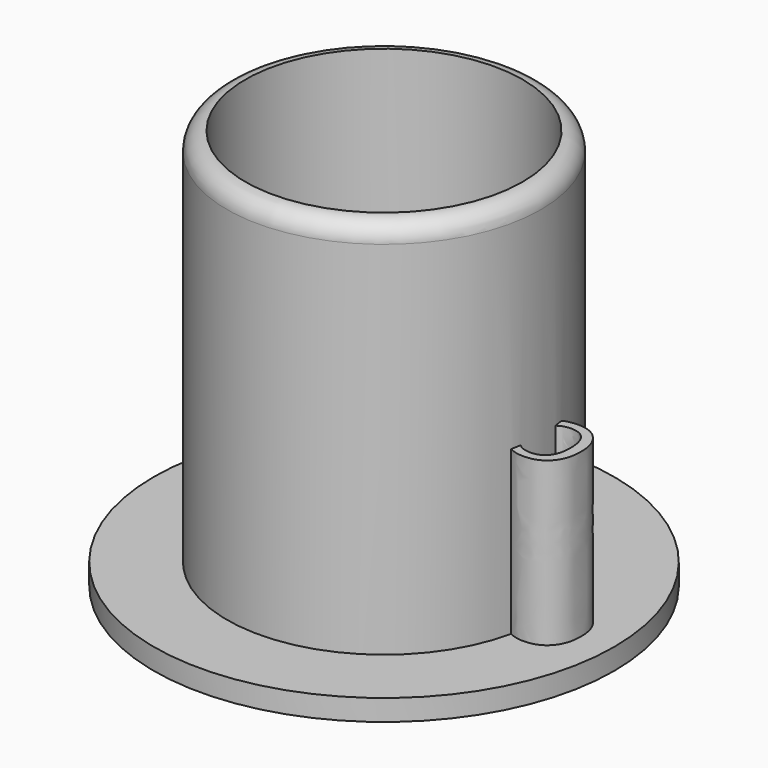
from build123d import *

# Parameters (mm, degrees)
F0_R     = 43.4000447198
F1_DEPTH = 110.744
F2_T     = -5.08
F3_R     = 63.6187489092
F4_DEPTH = 5.842
F5_R     = 5.07999
F6_W     = 2.7671808675
F6_H     = 25.928324776
F7_DEPTH = 50.8


# Not quite as in the source:
# - a fillet or chamfer is up to 0.001 mm smaller than in the source, because OpenCascade refuses the exact size


with BuildPart() as f1:
    # F0 (on Top) → F1 (new body)
    with BuildSketch(Plane.XY):
        Circle(F0_R)
    extrude(amount=F1_DEPTH)

    # F2
    f2_openings = [f1.faces().sort_by_distance(p)[0] for p in [
        (0, 0, 110.744),
    ]]
    offset(amount=F2_T, openings=f2_openings)

    # F3 (on Top) → F4 (join)
    with BuildSketch(Plane.XY):
        Circle(F3_R)
    extrude(amount=F4_DEPTH)

    # F5 (radius 5.08 in the source; OpenCascade refuses exactly that, so slightly less here)
    f5_edges = [f1.edges().sort_by_distance(p)[0] for p in [
        (-43.400045, 0, 110.744),
    ]]
    fillet(f5_edges, radius=F5_R)

    # F6 (on Top) → F7 (join)
    with BuildSketch(Plane.XY):
        with BuildLine():
            ThreePointArc((22.0028883346, -9.7789997235), (23.5536000152, -4.9983854371), (24.0781214104, 0))
            ThreePointArc((24.0781214104, 0), (23.5424460635, 5.0506597592), (21.9592547789, 9.8765915281))
            Line((21.9592547789, 9.8765915281), (21.9592547789, -9.7789997235))
            Line((21.9592547789, -9.7789997235), (22.0028883346, -9.7789997235))
        make_face()
        with BuildLine():
            ThreePointArc((21.9592547789, 9.8765915281), (23.5424460635, 5.0506597592), (24.0781214104, 0))
            ThreePointArc((24.0781214104, 0), (23.5536000152, -4.9983854371), (22.0028883346, -9.7789997235))
            Line((22.0028883346, -9.7789997235), (24.7264356464, -9.7789997235))
            Line((24.7264356464, -9.7789997235), (24.7264356464, 16.1493250525))
            Line((24.7264356464, 16.1493250525), (21.9592547789, 16.1493250525))
            Line((21.9592547789, 16.1493250525), (21.9592547789, 9.8765915281))
        make_face()
        with BuildLine():
            Line((21.9592547789, -9.7789997235), (21.9592547789, 9.8765915281))
            ThreePointArc((21.9592547789, 9.8765915281), (2.7373131328, 23.9220201377), (-19.1605677938, 14.5817890698))
            Line((-19.1605677938, 14.5817890698), (-19.1165860754, 14.5817890698))
            Line((-19.1165860754, 14.5817890698), (-19.1165860754, 4.2168572654))
            Line((-19.1165860754, 4.2168572654), (-6.283051686, 4.2168572654))
            Line((-6.283051686, 4.2168572654), (-6.283051686, 14.5817890698))
            Line((-6.283051686, 14.5817890698), (-3.4518897579, 14.5817890698))
            Line((-3.4518897579, 14.5817890698), (-3.4518897579, -9.7789997235))
            Line((-3.4518897579, -9.7789997235), (-6.283051686, -9.7789997235))
            Line((-6.283051686, -9.7789997235), (-6.283051686, 1.6842736198))
            Line((-6.283051686, 1.6842736198), (-19.1165860754, 1.6842736198))
            Line((-19.1165860754, 1.6842736198), (-19.1165860754, -9.7789997235))
            Line((-19.1165860754, -9.7789997235), (-21.9477480035, -9.7789997235))
            Line((-21.9477480035, -9.7789997235), (-21.9477480035, 9.9021355389))
            ThreePointArc((-21.9477480035, 9.9021355389), (-9.8406062526, -21.9754044158), (22.0028883346, -9.7789997235))
            Line((22.0028883346, -9.7789997235), (21.9592547789, -9.7789997235))
        make_face()
        with BuildLine():
            add(Edge.make_bspline(
                [(13.6843709515, -9.837649029), (12.3780909659, -10.1149002912), (10.5279719658, -10.1149002912)],
                knots=[0, 0, 0, 1, 1, 1], degree=2))
            add(Edge.make_bspline(
                [(10.5279719658, -10.1149002912), (6.4811698879, -10.1149002912), (4.1378635463, -7.6462977061)],
                knots=[0, 0, 0, 1, 1, 1], degree=2))
            add(Edge.make_bspline(
                [(4.1378635463, -7.6462977061), (1.7945572048, -5.177695121), (1.7945572048, -0.8003242304)],
                knots=[0, 0, 0, 1, 1, 1], degree=2))
            add(Edge.make_bspline(
                [(1.7945572048, -0.8003242304), (1.7945572048, 3.6197007006), (3.9699132625, 6.2189312842)],
                knots=[0, 0, 0, 1, 1, 1], degree=2))
            add(Edge.make_bspline(
                [(3.9699132625, 6.2189312842), (6.1452693202, 8.8181618679), (9.81351679, 8.8181618679)],
                knots=[0, 0, 0, 1, 1, 1], degree=2))
            add(Edge.make_bspline(
                [(9.81351679, 8.8181618679), (13.2418352829, 8.8181618679), (15.2412434242, 6.560163607)],
                knots=[0, 0, 0, 1, 1, 1], degree=2))
            add(Edge.make_bspline(
                [(15.2412434242, 6.560163607), (17.2406515655, 4.3021653461), (17.2406515655, 0.601927346)],
                knots=[0, 0, 0, 1, 1, 1], degree=2))
            Line((17.2406515655, 0.601927346), (17.2406515655, -1.1468883082))
            Line((17.2406515655, -1.1468883082), (4.6630414181, -1.1468883082))
            add(Edge.make_bspline(
                [(4.6630414181, -1.1468883082), (4.7483494988, -4.3619365994), (6.2892267063, -6.0281100505)],
                knots=[0, 0, 0, 1, 1, 1], degree=2))
            add(Edge.make_bspline(
                [(6.2892267063, -6.0281100505), (7.8301039139, -7.6942835015), (10.6292753117, -7.6942835015)],
                knots=[0, 0, 0, 1, 1, 1], degree=2))
            add(Edge.make_bspline(
                [(10.6292753117, -7.6942835015), (13.5777358507, -7.6942835015), (16.4568835741, -6.4626480865)],
                knots=[0, 0, 0, 1, 1, 1], degree=2))
            Line((16.4568835741, -6.4626480865), (16.4568835741, -8.9312506716))
            add(Edge.make_bspline(
                [(16.4568835741, -8.9312506716), (14.9906509372, -9.5603977667), (13.6843709515, -9.837649029)],
                knots=[0, 0, 0, 1, 1, 1], degree=2))
        make_face(mode=Mode.SUBTRACT)
        with BuildLine():
            Line((-19.1165860754, 14.5817890698), (-19.1605677938, 14.5817890698))
            ThreePointArc((-19.1605677938, 14.5817890698), (-20.6869088124, 12.3210281406), (-21.9477480035, 9.9021355389))
            Line((-21.9477480035, 9.9021355389), (-21.9477480035, -9.7789997235))
            Line((-21.9477480035, -9.7789997235), (-19.1165860754, -9.7789997235))
            Line((-19.1165860754, -9.7789997235), (-19.1165860754, 1.6842736198))
            Line((-19.1165860754, 1.6842736198), (-6.283051686, 1.6842736198))
            Line((-6.283051686, 1.6842736198), (-6.283051686, -9.7789997235))
            Line((-6.283051686, -9.7789997235), (-3.4518897579, -9.7789997235))
            Line((-3.4518897579, -9.7789997235), (-3.4518897579, 14.5817890698))
            Line((-3.4518897579, 14.5817890698), (-6.283051686, 14.5817890698))
            Line((-6.283051686, 14.5817890698), (-6.283051686, 4.2168572654))
            Line((-6.283051686, 4.2168572654), (-19.1165860754, 4.2168572654))
            Line((-19.1165860754, 4.2168572654), (-19.1165860754, 14.5817890698))
        make_face()
        with BuildLine():
            ThreePointArc((-21.9477480035, 9.9021355389), (-20.6869088124, 12.3210281406), (-19.1605677938, 14.5817890698))
            Line((-19.1605677938, 14.5817890698), (-21.9477480035, 14.5817890698))
            Line((-21.9477480035, 14.5817890698), (-21.9477480035, 9.9021355389))
        make_face()
        with Locations((31.9749566279, 3.1851626645)):
            Rectangle(F6_W, F6_H)
        with BuildLine():
            add(Edge.make_bspline(
                [(54.9841455177, -0.629708069), (54.9841455177, -5.0977187954), (52.7368107669, -7.6063095433)],
                knots=[0, 0, 0, 1, 1, 1], degree=2))
            add(Edge.make_bspline(
                [(52.7261472568, 6.2669170796), (54.9841455177, 3.7156722913), (54.9841455177, -0.629708069)],
                knots=[0, 0, 0, 1, 1, 1], degree=2))
            add(Edge.make_bspline(
                [(46.6399488748, 8.8181618679), (50.4681489959, 8.8181618679), (52.7261472568, 6.2669170796)],
                knots=[0, 0, 0, 1, 1, 1], degree=2))
            add(Edge.make_bspline(
                [(40.4391177593, 6.3255663851), (42.6731231225, 8.8181618679), (46.6399488748, 8.8181618679)],
                knots=[0, 0, 0, 1, 1, 1], degree=2))
            add(Edge.make_bspline(
                [(38.2051123961, -0.629708069), (38.2051123961, 3.8329709023), (40.4391177593, 6.3255663851)],
                knots=[0, 0, 0, 1, 1, 1], degree=2))
            add(Edge.make_bspline(
                [(39.2394728745, -5.66288483), (38.2051123961, -3.5141875475), (38.2051123961, -0.629708069)],
                knots=[0, 0, 0, 1, 1, 1], degree=2))
            add(Edge.make_bspline(
                [(42.1719381484, -8.9632412019), (40.2738333529, -7.8115821125), (39.2394728745, -5.66288483)],
                knots=[0, 0, 0, 1, 1, 1], degree=2))
            add(Edge.make_bspline(
                [(46.5226502638, -10.1149002912), (44.0700429438, -10.1149002912), (42.1719381484, -8.9632412019)],
                knots=[0, 0, 0, 1, 1, 1], degree=2))
            add(Edge.make_bspline(
                [(52.7368107669, -7.6063095433), (50.4894760161, -10.1149002912), (46.5226502638, -10.1149002912)],
                knots=[0, 0, 0, 1, 1, 1], degree=2))
        make_face()
        with BuildLine():
            add(Edge.make_bspline(
                [(41.0735966094, -0.629708069), (41.0735966094, -4.1326711325), (42.4731823083, -5.9641289899)],
                knots=[0, 0, 0, 1, 1, 1], degree=2))
            add(Edge.make_bspline(
                [(42.4571870432, 4.6833858317), (41.0735966094, 2.8999137697), (41.0735966094, -0.629708069)],
                knots=[0, 0, 0, 1, 1, 1], degree=2))
            add(Edge.make_bspline(
                [(46.5546407941, 6.4668578937), (43.840777477, 6.4668578937), (42.4571870432, 4.6833858317)],
                knots=[0, 0, 0, 1, 1, 1], degree=2))
            add(Edge.make_bspline(
                [(50.7134097279, 4.659392934), (49.3058263964, 6.4668578937), (46.5546407941, 6.4668578937)],
                knots=[0, 0, 0, 1, 1, 1], degree=2))
            add(Edge.make_bspline(
                [(52.1209930594, -0.629708069), (52.1209930594, 2.8519279743), (50.7134097279, 4.659392934)],
                knots=[0, 0, 0, 1, 1, 1], degree=2))
            add(Edge.make_bspline(
                [(50.7134097279, -5.9721266225), (52.1209930594, -4.1486663977), (52.1209930594, -0.629708069)],
                knots=[0, 0, 0, 1, 1, 1], degree=2))
            add(Edge.make_bspline(
                [(46.5866313243, -7.7955868474), (49.3058263964, -7.7955868474), (50.7134097279, -5.9721266225)],
                knots=[0, 0, 0, 1, 1, 1], degree=2))
            add(Edge.make_bspline(
                [(42.4731823083, -5.9641289899), (43.8727680072, -7.7955868474), (46.5866313243, -7.7955868474)],
                knots=[0, 0, 0, 1, 1, 1], degree=2))
        make_face(mode=Mode.SUBTRACT)
    extrude(amount=F7_DEPTH)


solid = f1.part
